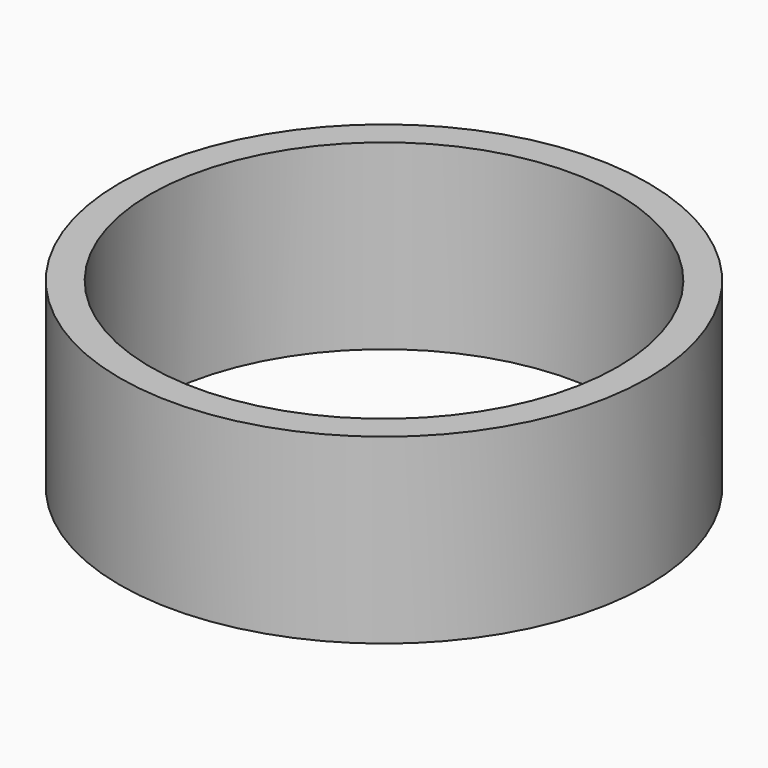
from build123d import *

# Parameters (mm, degrees)
F0_R     = 21.75
F0_R_2   = 19.25
F1_DEPTH = 15


# Not quite as in the source:
# - a feature names something its author has since deleted; it is built from what else it names


with BuildPart() as f1:
    # F0 (on Top) → F1 (new body)
    with BuildSketch(Plane.XY):
        Circle(F0_R)
        Circle(F0_R_2, mode=Mode.SUBTRACT)
    extrude(amount=F1_DEPTH)


solid = f1.part
